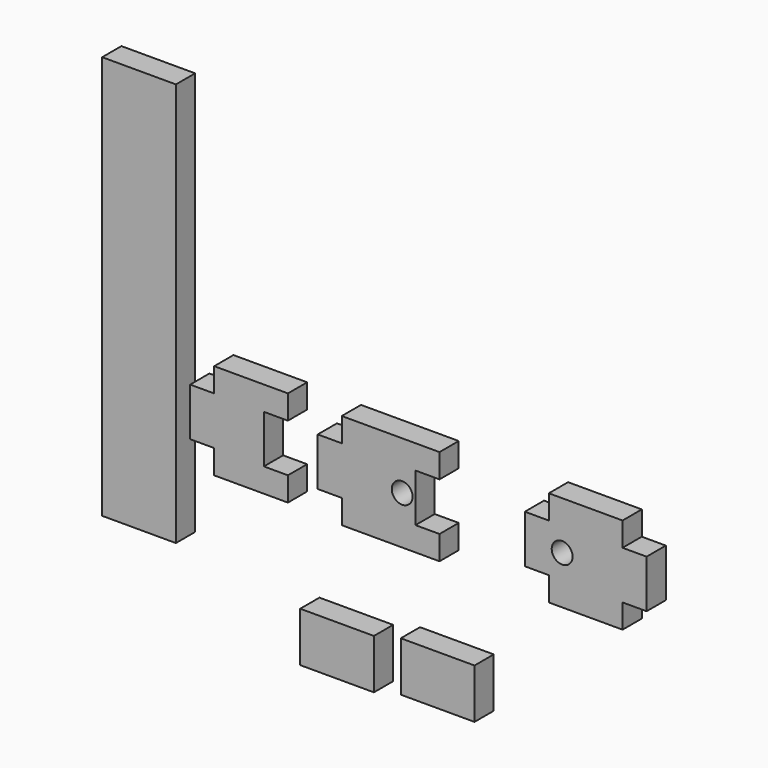
from build123d import *

# Parameters (mm, degrees)
F1_DEPTH = 19.05
F0_R     = 8.255
F0_W     = 58.42
F0_H     = 39.37
F0_H_2   = 320.04
F2_DEPTH = 19.05


# Not quite as in the source:
# - a feature names something its author has since deleted; it is built from what else it names


with BuildPart() as f1:
    # F0 (on Front) → F1 (new body)
    with BuildSketch(Plane.XZ):
        Polygon((-84.963388741, 46.6005802155), (-143.383388741, 46.6005802155), (-143.383388741, 27.5505802155), (-162.433388741, 27.5505802155), (-162.433388741, -10.5494197845), (-143.383388741, -10.5494197845), (-143.383388741, -29.5994197845), (-84.963388741, -29.5994197845), (-84.963388741, -10.5494197845), (-104.013388741, -10.5494197845), (-104.013388741, 27.5505802155), (-84.963388741, 27.5505802155), align=None)
    extrude(amount=F1_DEPTH)


with BuildPart() as f1b:
    # F0 (on Front) → F1, piece 2 (new body)
    with BuildSketch(Plane.XZ):
        Polygon((35.1907358062, 44.7134936616), (-42.2792641938, 44.7134936616), (-42.2792641938, 25.6634936616), (-61.3292641938, 25.6634936616), (-61.3292641938, -12.4365063384), (-42.2792641938, -12.4365063384), (-42.2792641938, -31.4865063384), (35.1907358062, -31.4865063384), (35.1907358062, -12.4365063384), (16.1407358062, -12.4365063384), (16.1407358062, 25.6634936616), (35.1907358062, 25.6634936616), align=None)
        with Locations((5.5997358062, 6.6134936616)):
            Circle(F0_R, mode=Mode.SUBTRACT)
    extrude(amount=F1_DEPTH)


with BuildPart() as f1c:
    # F0 (on Front) → F1, piece 3 (new body)
    with BuildSketch(Plane.XZ):
        Polygon((180.2678704262, 44.1764993489), (121.8478704262, 44.1764993489), (121.8478704262, 25.1264993489), (102.7978704262, 25.1264993489), (102.7978704262, -12.9735006511), (121.8478704262, -12.9735006511), (121.8478704262, -32.0235006511), (180.2678704262, -32.0235006511), (180.2678704262, -12.9735006511), (199.3178704262, -12.9735006511), (199.3178704262, 25.1264993489), (180.2678704262, 25.1264993489), align=None)
        with Locations((132.3888704262, 6.0764993489)):
            Circle(F0_R, mode=Mode.SUBTRACT)
    extrude(amount=F1_DEPTH)


with BuildPart() as f1d:
    # F0 (on Front) → F1, piece 4 (new body)
    with BuildSketch(Plane.XZ):
        with Locations((-46.0048330212, -120.1514003849)):
            Rectangle(F0_W, F0_H)
    extrude(amount=F1_DEPTH)


with BuildPart() as f1e:
    # F0 (on Front) → F1, piece 5 (new body)
    with BuildSketch(Plane.XZ):
        with Locations((33.7117160036, -114.8489843512)):
            Rectangle(F0_W, F0_H)
    extrude(amount=F1_DEPTH)


with BuildPart() as f2:
    # F0 (on Front) → F2 (new body)
    with BuildSketch(Plane.XZ):
        with Locations((-202.9565411425, 73.3008670402)):
            Rectangle(F0_W, F0_H_2)
    extrude(amount=F2_DEPTH)


solid = Compound([f1.part, f1b.part, f1c.part, f1d.part, f1e.part, f2.part])
